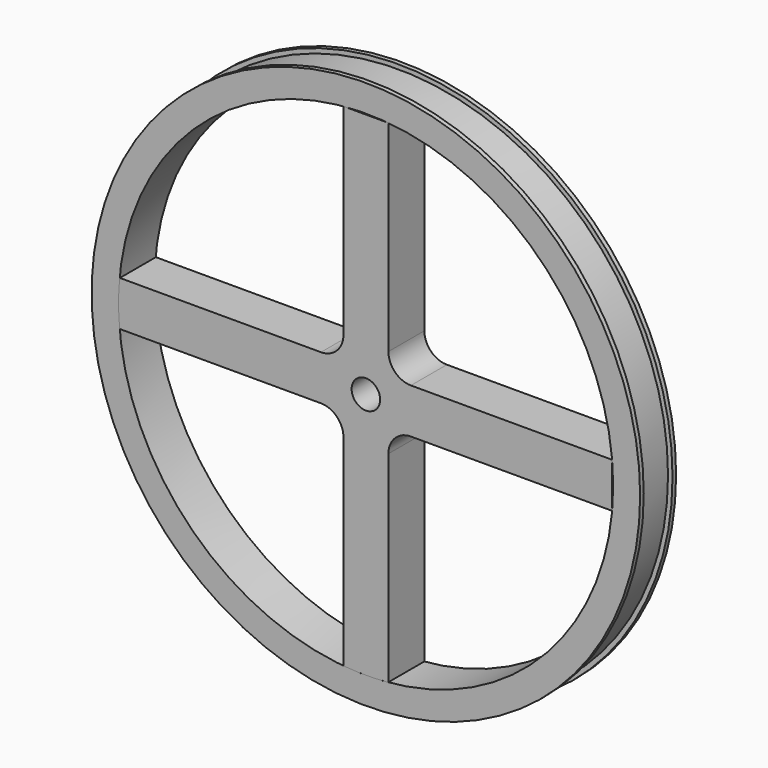
from build123d import *

# Parameters (mm, degrees)
F0_R      = 76.2
F2_DEPTH  = 12.7
F3_R      = 77.47
F4_DEPTH  = 1.27
F5_R      = 77.47
F6_DEPTH  = 1.27
F7_R      = 4.0259
F8_DEPTH  = 25.4
F1_R      = 69.85
F10_DEPTH = 25.4
F11_R     = 6.35
F12_DEPTH = 12.7
F13_DEPTH = 25.4
F15_DEPTH = 12.7
F16_DEPTH = 25.4


# Not quite as in the source:
# - the program builds the solid bodies; features that only make, move or delete a surface that nothing else refers to are left out


with BuildPart() as f2:
    # F0 (on Front) → F2 (new body)
    with BuildSketch(Plane.XZ):
        with Locations((-22.4455539137, 18.7809728086)):
            Circle(F0_R)
    extrude(amount=F2_DEPTH)

    # F3 (on face) → F4 (join)
    with BuildSketch(Plane.XZ.offset(12.7)):
        with Locations((-22.4455539137, 18.7809728086)):
            Circle(F3_R)
    extrude(amount=-F4_DEPTH)

    # F5 (on face) → F6 (join)
    with BuildSketch(Plane.XZ):
        with Locations((-22.4455539137, 18.7809728086)):
            Circle(F5_R)
    extrude(amount=F6_DEPTH)

    # F7 (on face) → F8 (cut)
    with BuildSketch(Plane.XZ):
        with Locations((-22.4455539137, 18.7809728086)):
            Circle(F7_R)
    extrude(amount=F8_DEPTH, mode=Mode.SUBTRACT)

    # F1 (on face) → F10 (cut)
    with BuildSketch(Plane.XZ):
        with Locations((-22.4455539137, 18.7809728086)):
            Circle(F1_R)
    extrude(amount=F10_DEPTH, mode=Mode.SUBTRACT)


with BuildPart() as f12:
    # F11 (on face) → F12 (new body)
    with BuildSketch(Plane.XZ):
        with Locations((-22.4455539137, 18.7809728086)):
            Circle(F11_R)
    extrude(amount=F12_DEPTH)

    # F7 (on face) → F13 (cut)
    with BuildSketch(Plane.XZ):
        with Locations((-22.4455539137, 18.7809728086)):
            Circle(F7_R)
    extrude(amount=F13_DEPTH, mode=Mode.SUBTRACT)


with BuildPart() as f15:
    # F14 (on face) → F15 (new body)
    with BuildSketch(Plane.XZ.offset(12.7)):
        with BuildLine():
            Line((-16.083676368, -50.7787067054), (-16.083676368, -44.7071496457))
            Line((-16.083676368, -44.7071496457), (-16.083676368, 6.0809728086))
            ThreePointArc((-16.083676368, 6.0809728086), (-14.2238044285, 10.5711008691), (-9.733676368, 12.4309728086))
            Line((-9.733676368, 12.4309728086), (47.1152108894, 12.4309728086))
            Line((47.1152108894, 12.4309728086), (47.1152108894, 25.1309728086))
            Line((47.1152108894, 25.1309728086), (-9.733676368, 25.1309728086))
            ThreePointArc((-9.733676368, 25.1309728086), (-14.2238044285, 26.9908447481), (-16.083676368, 31.4809728086))
            Line((-16.083676368, 31.4809728086), (-16.083676368, 82.2690952629))
            Line((-16.083676368, 82.2690952629), (-16.083676368, 88.3406523226))
            Line((-16.083676368, 88.3406523226), (-28.7868808955, 88.3425288012))
            Line((-28.7868808955, 88.3425288012), (-28.7868808955, 31.4809728086))
            ThreePointArc((-28.7868808955, 31.4809728086), (-30.646752835, 26.9908447481), (-35.1368808955, 25.1309728086))
            Line((-35.1368808955, 25.1309728086), (-92.0063187169, 25.1309728086))
            ThreePointArc((-92.0063187169, 25.1309728086), (-92.2955539137, 18.7809728086), (-92.0063187169, 12.4309728086))
            Line((-92.0063187169, 12.4309728086), (-35.1368808955, 12.4309728086))
            ThreePointArc((-35.1368808955, 12.4309728086), (-30.646752835, 10.5711008691), (-28.7868808955, 6.0809728086))
            Line((-28.7868808955, 6.0809728086), (-28.7868808955, -50.780583184))
            ThreePointArc((-28.7868808955, -50.780583184), (-22.4352358852, -51.0690264293), (-16.083676368, -50.7787067054))
        make_face()
    extrude(amount=-F15_DEPTH)

    # F7 (on face) → F16 (cut)
    with BuildSketch(Plane.XZ):
        with Locations((-22.4455539137, 18.7809728086)):
            Circle(F7_R)
    extrude(amount=F16_DEPTH, mode=Mode.SUBTRACT)


solid = Compound([f2.part, f12.part, f15.part])
